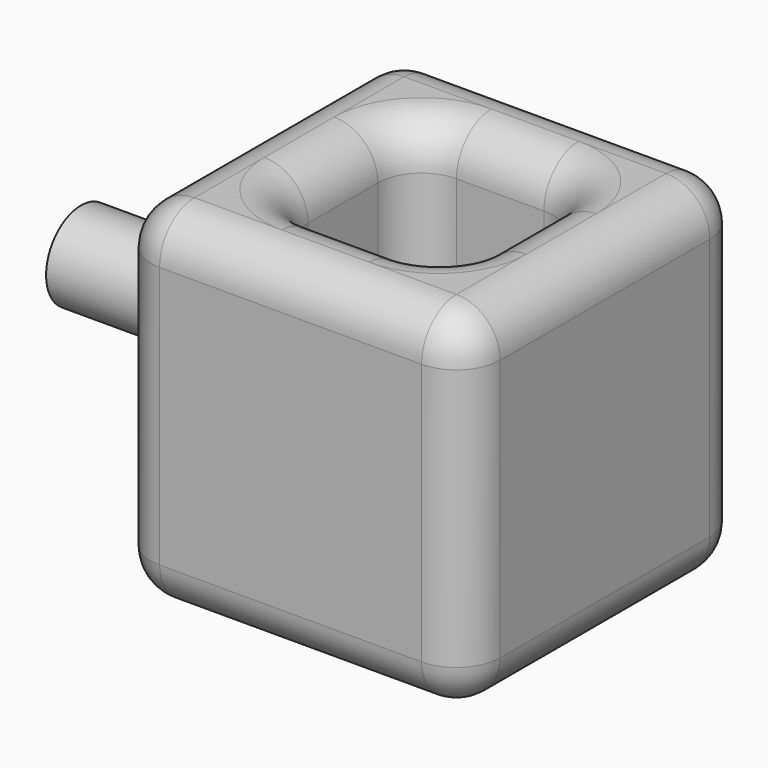
from build123d import *

# Parameters (mm, degrees)
F0_W     = 50.8
F0_H     = 50.8
F1_DEPTH = 50.8
F2_T     = -12.7
F3_R     = 6.35
F4_DEPTH = 25.4
F5_R     = 6.34999


# Not quite as in the source:
# - a fillet or chamfer is up to 0.001 mm smaller than in the source, because OpenCascade refuses the exact size


with BuildPart() as f1:
    # F0 (on Right) → F1 (new body)
    with BuildSketch(Plane.YZ):
        Rectangle(F0_W, F0_H)
    extrude(amount=F1_DEPTH)

    # F2
    f2_openings = [f1.faces().sort_by_distance(p)[0] for p in [
        (25.4, 0, 25.4),
        (25.4, 0, -25.4),
    ]]
    offset(amount=F2_T, openings=f2_openings)

    # F3 (on face) → F4 (join)
    with BuildSketch(Plane(origin=(0, 0, 0), x_dir=(0, -1, 0), z_dir=(-1, 0, 0))):
        Circle(F3_R)
    extrude(amount=F4_DEPTH)

    # F5 (radius 6.35 in the source; OpenCascade refuses exactly that, so slightly less here)
    f5_edges = [f1.edges().sort_by_distance(p)[0] for p in [
        (50.8, -25.4, 0),
        (0, -25.4, 0),
        (50.8, 25.4, 0),
        (0, 25.4, 0),
        (12.7, -12.7, 0),
        (38.1, 12.7, 0),
        (12.7, 12.7, 0),
        (38.1, -12.7, 0),
        (25.4, 25.4, 25.4),
        (50.8, 0, 25.4),
        (25.4, -25.4, 25.4),
        (0, 0, 25.4),
        (25.4, 12.7, 25.4),
        (12.7, 0, 25.4),
        (25.4, -12.7, 25.4),
        (38.1, 0, 25.4),
        (25.4, -25.4, -25.4),
        (50.8, 0, -25.4),
        (25.4, 25.4, -25.4),
        (0, 0, -25.4),
        (25.4, -12.7, -25.4),
        (12.7, 0, -25.4),
        (25.4, 12.7, -25.4),
        (38.1, 0, -25.4),
    ]]
    fillet(f5_edges, radius=F5_R)


solid = f1.part
